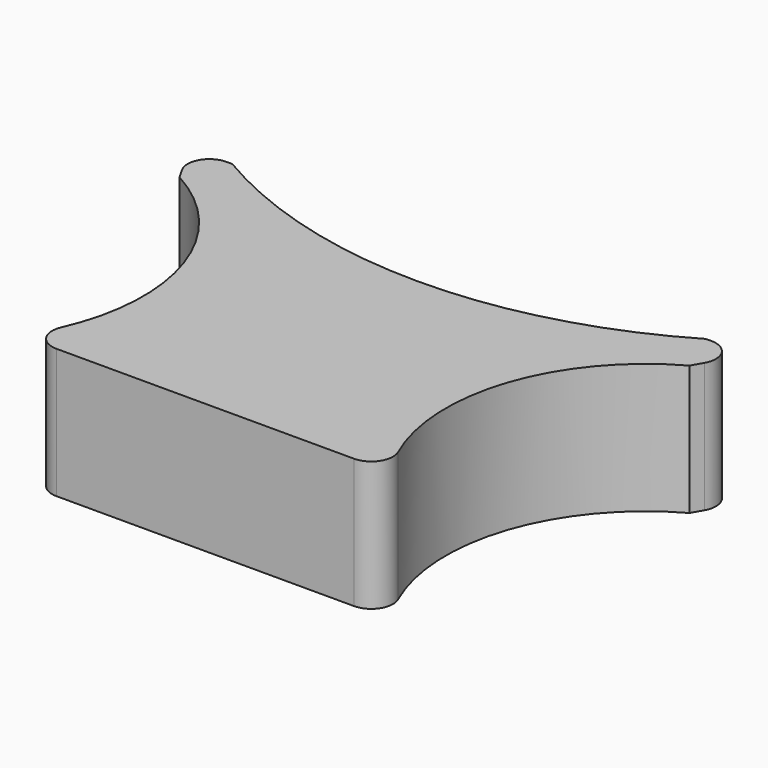
from build123d import *

# Parameters (mm, degrees)
F1_DEPTH = 3
F2_R     = 1


# Not quite as in the source:
# - a feature names something its author has since deleted; it is built from what else it names


with BuildPart() as f1:
    # F0 (on Top) → F1 (new body, symmetric)
    with BuildSketch(Plane.XY):
        with BuildLine():
            Line((-12.9470113486, 10.248668018), (-11.7864680784, 8.248668018))
            ThreePointArc((-11.7864680784, 8.248668018), (-7.2595115052, 2.3329471863), (-8.5698451786, -5))
            Line((-8.5698451786, -5), (8.5698451786, -5))
            ThreePointArc((8.5698451786, -5), (7.2595115052, 2.3329471863), (11.7864680784, 8.248668018))
            Line((11.7864680784, 8.248668018), (12.9470113486, 10.248668018))
            Line((12.9470113486, 10.248668018), (10.9470113486, 10.248668018))
            ThreePointArc((10.9470113486, 10.248668018), (0, 7.2662124228), (-10.9470113486, 10.248668018))
            Line((-10.9470113486, 10.248668018), (-12.9470113486, 10.248668018))
        make_face()
    extrude(amount=F1_DEPTH, both=True)

    # F2
    f2_edges = [f1.edges().sort_by_distance(p)[0] for p in [
        (-12.947011, 10.248668, 0),
        (12.947011, 10.248668, 0),
        (-8.569845, -5, 0),
        (8.569845, -5, 0),
    ]]
    fillet(f2_edges, radius=F2_R)


solid = f1.part
